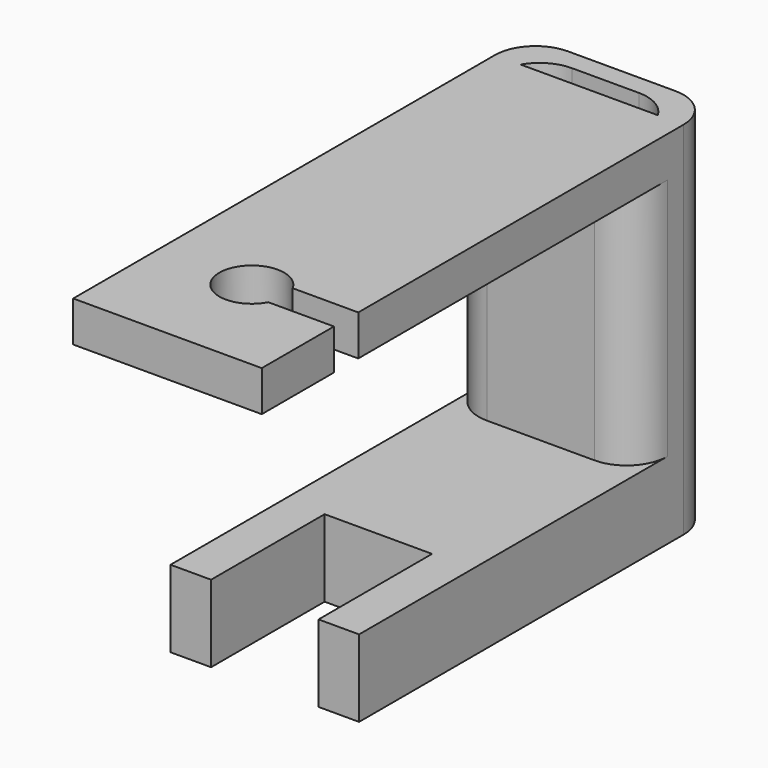
from build123d import *

# Parameters (mm, degrees)
F1_DEPTH  = 5.842
F2_DEPTH  = 5.08
F3_W      = 18.542
F3_H      = 5.08
F4_DEPTH  = 35.56
F5_W      = 18.542
F5_H      = 5.08
F6_DEPTH  = 58.42
F8_DEPTH  = 2.54
F9_DEPTH  = 2.54
F7_W      = 19.7188566824
F7_H      = 3.81
F10_DEPTH = 25.4
F11_DEPTH = 3.81
F12_DEPTH = 5.08
F13_DEPTH = 7.62
F14_W     = 18.542
F14_H     = 5.08
F15_DEPTH = 127
F16_R     = 5.07999
F18_DEPTH = 2.54
F19_W     = 5.08
F19_H     = 12.7
F20_DEPTH = 5.08


# Not quite as in the source:
# - two fillets or chamfers of one size are made in one step
# - a fillet or chamfer is up to 0.001 mm smaller than in the source, because OpenCascade refuses the exact size


with BuildPart() as f1:
    # F0 (on Top) → F1 (new body)
    with BuildSketch(Plane.XY):
        Polygon((-9.271, 43.18), (-9.271, 0), (-6.731, 0), (-6.731, 12.7), (6.731, 12.7), (6.731, 0), (9.271, 0), (9.271, 43.18), align=None)
    extrude(amount=F1_DEPTH)

    # F2 (add): a face of the model
    f2_faces = [f1.faces().sort_by_distance(p)[0] for p in [
        (0, 43.18, 2.921),
    ]]
    extrude(f2_faces, amount=F2_DEPTH)

    # F3 (on face) → F4 (join)
    with BuildSketch(Plane.XY.offset(5.842)):
        with Locations((0, 45.72)):
            Rectangle(F3_W, F3_H)
    extrude(amount=F4_DEPTH)

    # F5 (on face) → F6 (join)
    with BuildSketch(Plane.XZ.offset(-43.18)):
        with Locations((0, 38.862)):
            Rectangle(F5_W, F5_H)
    extrude(amount=F6_DEPTH)

    # F8 (add): a face of the model
    f8_faces = [f1.faces().sort_by_distance(p)[0] for p in [
        (-9.271, 0.7580485211, 2.921),
    ]]
    extrude(f8_faces, amount=F8_DEPTH)

    # F9 (add): a face of the model
    f9_faces = [f1.faces().sort_by_distance(p)[0] for p in [
        (9.271, 0.7580485211, 2.921),
    ]]
    extrude(f9_faces, amount=F9_DEPTH)

    # F7 (on face) → F10 (cut)
    with BuildSketch(Plane.XY.offset(41.402)):
        with BuildLine():
            ThreePointArc((3.5898566824, -0.127), (3.9436831489, -1.0504404137), (4.064, -2.032))
            ThreePointArc((4.064, -2.032), (3.9436831489, -3.0135595863), (3.5898566824, -3.937))
            Line((3.5898566824, -3.937), (9.271, -3.937))
            Line((9.271, -3.937), (9.271, -0.127))
            Line((9.271, -0.127), (3.5898566824, -0.127))
        make_face()
        with BuildLine():
            Line((3.5898566824, -3.937), (3.5898566824, -0.127))
            ThreePointArc((3.5898566824, -0.127), (-4.064, -2.032), (3.5898566824, -3.937))
        make_face()
        with BuildLine():
            ThreePointArc((3.5898566824, -3.937), (3.9436831489, -3.0135595863), (4.064, -2.032))
            ThreePointArc((4.064, -2.032), (3.9436831489, -1.0504404137), (3.5898566824, -0.127))
            Line((3.5898566824, -0.127), (3.5898566824, -3.937))
        make_face()
        with Locations((19.1304283412, -2.032)):
            Rectangle(F7_W, F7_H)
    extrude(amount=-F10_DEPTH, mode=Mode.SUBTRACT)

    # F11 (add): a face of the model
    f11_faces = [f1.faces().sort_by_distance(p)[0] for p in [
        (0, 27.2669507324, 0),
    ]]
    extrude(f11_faces, amount=F11_DEPTH)

    # F12 (cut): a face of the model
    f12_faces = [f1.faces().sort_by_distance(p)[0] for p in [
        (0, 12.7, 1.016),
    ]]
    extrude(f12_faces, amount=-F12_DEPTH, mode=Mode.SUBTRACT)

    # F13 (add): a face of the model
    f13_faces = [f1.faces().sort_by_distance(p)[0] for p in [
        (0, 48.26, 18.796),
    ]]
    extrude(f13_faces, amount=F13_DEPTH)

    # F14 (on face) → F15 (cut)
    with BuildSketch(Plane.XY.offset(41.402)):
        with Locations((0, 50.8)):
            Rectangle(F14_W, F14_H)
    extrude(amount=-F15_DEPTH, mode=Mode.SUBTRACT)

    # F16 (radius 5.08 in the source; OpenCascade refuses exactly that, so slightly less here)
    f16_edges = [f1.edges().sort_by_distance(p)[0] for p in [
        (9.271, 53.34, 18.796),
        (-9.271, 53.34, 18.796),
        (-11.811, 55.88, 18.796),
        (-11.811, 43.18, 21.082),
        (11.811, 43.18, 21.082),
        (11.811, 55.88, 18.796),
    ]]
    fillet(f16_edges, radius=F16_R)

    # F18 (add): a face of the model
    f18_faces = [f1.faces().sort_by_distance(p)[0] for p in [
        (0, 48.26, 18.796),
    ]]
    extrude(f18_faces, amount=F18_DEPTH)

    # F19 (on face) → F20 (cut)
    with BuildSketch(Plane(origin=(0, 55.88, 0), x_dir=(-1, 0, 0), z_dir=(0, 1, 0))):
        with Locations((0.127, 19.812)):
            Rectangle(F19_W, F19_H)
    extrude(amount=-F20_DEPTH, mode=Mode.SUBTRACT)


solid = f1.part
